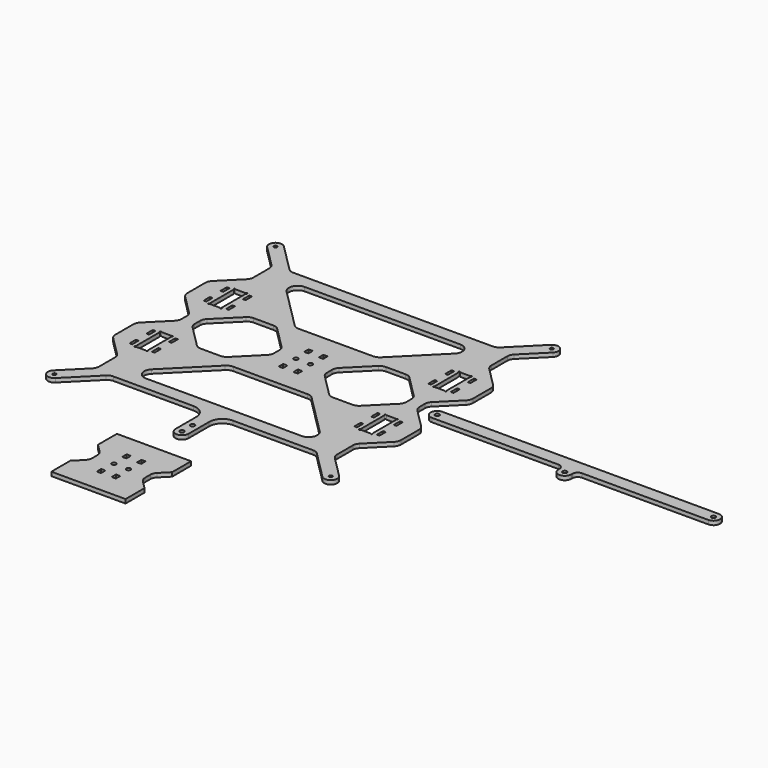
from build123d import *

# Parameters (mm, degrees)
F0_R     = 1.25
F0_W     = 2
F0_H     = 6
F0_R_2   = 1.6
F0_W_2   = 3.2
F0_H_2   = 4.2
F1_DEPTH = 3
F2_R     = 1.6
F3_DEPTH = 3
F6_R     = 1.25
F6_R_2   = 1.6
F6_W     = 2
F6_H     = 6
F7_DEPTH = 25


# Not quite as in the source:
# - ends of sketch curves that miss each other by under 0.0002 mm in the source are joined


with BuildPart() as f1:
    # F0 (on Top) → F1 (new body)
    with BuildSketch(Plane.XY):
        with BuildLine():
            ThreePointArc((-90.000032, 74.332551), (-90.4567550164, 72.0364496965), (-91.7573921058, 70.0899091058))
            Line((-91.7573921058, 70.0899091058), (-106.242677, 55.604628))
            ThreePointArc((-106.242677, 55.604628), (-107.5433139836, 53.6580873035), (-108.000037, 51.361986))
            Line((-108.000037, 51.361986), (-108.000037, 34.332561))
            ThreePointArc((-108.000037, 34.332561), (-107.5433139836, 32.0364596965), (-106.2426768942, 30.0899191058))
            Line((-106.2426768942, 30.0899191058), (-91.757392, 15.604638))
            ThreePointArc((-91.757392, 15.604638), (-90.4567550164, 13.6580973035), (-90.000032, 11.361996))
            Line((-90.000032, 11.361996), (-90.000032, 6.332547))
            ThreePointArc((-90.000032, 6.332547), (-90.4567550164, 4.0364456965), (-91.7573921058, 2.0899051058))
            Line((-91.7573921058, 2.0899051058), (-106.242677, -12.395376))
            ThreePointArc((-106.242677, -12.395376), (-107.5433139836, -14.3419166965), (-108.000037, -16.638018))
            Line((-108.000037, -16.638018), (-108.000037, -33.667443))
            ThreePointArc((-108.000037, -33.667443), (-107.5433139836, -35.9635443035), (-106.2426768942, -37.9100848942))
            Line((-106.2426768942, -37.9100848942), (-91.757392, -52.395366))
            ThreePointArc((-91.757392, -52.395366), (-90.4567550164, -54.3419066965), (-90.000032, -56.638008))
            Line((-90.000032, -56.638008), (-90.000032, -71.667432))
            ThreePointArc((-90.000032, -71.667432), (-90.4567550164, -73.9635333035), (-91.7573921058, -75.9100738942))
            Line((-91.7573921058, -75.9100738942), (-108.000037, -92.15271))
            ThreePointArc((-108.000037, -92.15271), (-108.0000399189, -99.1527094189), (-101.0000403311, -99.1527116689))
            Line((-101.0000403311, -99.1527116689), (-79.75736, -77.910043))
            ThreePointArc((-79.75736, -77.910043), (-77.8108196502, -76.6094067458), (-75.514719, -76.152684))
            Line((-75.514719, -76.152684), (-14.949747, -76.152684))
            ThreePointArc((-14.949747, -76.152684), (-7.8786791881, -79.0816161881), (-4.949747, -86.152684))
            Line((-4.949747, -86.152684), (-4.949747, -105.652688))
            ThreePointArc((-4.949747, -105.652688), (0, -110.602435), (4.949747, -105.652688))
            Line((4.949747, -105.652688), (4.949747, -86.152684))
            ThreePointArc((4.949747, -86.152684), (7.8786791881, -79.0816161881), (14.949747, -76.152684))
            Line((14.949747, -76.152684), (75.51472, -76.152684))
            ThreePointArc((75.51472, -76.152684), (77.8108203236, -76.6094066105), (79.7573603942, -77.9100426058))
            Line((79.7573603942, -77.9100426058), (101.00004, -99.152712))
            ThreePointArc((101.00004, -99.152712), (108.0000396689, -99.1527096689), (108.0000376689, -92.1527103311))
            Line((108.0000376689, -92.1527103311), (91.757322, -75.910003))
            ThreePointArc((91.757322, -75.910003), (90.4566842869, -73.9634619568), (89.999961, -71.66736))
            Line((89.999961, -71.66736), (89.999961, -56.638066))
            ThreePointArc((89.999961, -56.638066), (90.4566823928, -54.3419686162), (91.7573151058, -52.3954301058))
            Line((91.7573151058, -52.3954301058), (106.242579, -37.910128))
            ThreePointArc((106.242579, -37.910128), (107.5432106505, -35.9635916935), (107.999933, -33.667497))
            Line((107.999933, -33.667497), (107.999947, -16.638072))
            ThreePointArc((107.999947, -16.638072), (107.5432260227, -14.3419706193), (106.2425908942, -12.3954291058))
            Line((106.2425908942, -12.3954291058), (91.757319, 2.089867))
            ThreePointArc((91.757319, 2.089867), (90.4566842014, 4.036405465), (89.999962, 6.332504))
            Line((89.999962, 6.332504), (89.999961, 11.361951))
            ThreePointArc((89.999961, 11.361951), (90.4566847161, 13.6580559928), (91.7573251058, 15.6045988942))
            Line((91.7573251058, 15.6045988942), (106.242624, 30.089866))
            ThreePointArc((106.242624, 30.089866), (107.5432638092, 32.036405447), (107.999989, 34.332507))
            Line((107.999989, 34.332507), (108.000003, 51.361932))
            ThreePointArc((108.000003, 51.361932), (107.5432790462, 53.6580405668), (106.2426358942, 55.6045858942))
            Line((106.2426358942, 55.6045858942), (91.757328, 70.089844))
            ThreePointArc((91.757328, 70.089844), (90.4566857752, 72.0363864502), (89.999961, 74.332492))
            Line((89.999961, 74.332492), (89.999961, 89.361904))
            ThreePointArc((89.999961, 89.361904), (90.4566841517, 91.6580056302), (91.7573216058, 93.6045463942))
            Line((91.7573216058, 93.6045463942), (108.000038, 109.847254))
            ThreePointArc((108.000038, 109.847254), (108.0000394189, 116.8472529189), (101.0000403311, 116.8472546689))
            Line((101.0000403311, 116.8472546689), (79.757314, 95.60454))
            ThreePointArc((79.757314, 95.60454), (77.810773997, 94.3039044752), (75.514674, 93.847182))
            Line((75.514674, 93.847182), (-75.514673, 93.847182))
            ThreePointArc((-75.514673, 93.847182), (-77.8107733236, 94.3039046105), (-79.7573133942, 95.6045406058))
            Line((-79.7573133942, 95.6045406058), (-101.00004, 116.847255))
            ThreePointArc((-101.00004, 116.847255), (-108.0000396689, 116.8472526689), (-108.0000376689, 109.8472533311))
            Line((-108.0000376689, 109.8472533311), (-91.757392, 93.604617))
            ThreePointArc((-91.757392, 93.604617), (-90.4567550164, 91.6580763035), (-90.000032, 89.361975))
            Line((-90.000032, 89.361975), (-90.000032, 74.332551))
        make_face()
        with Locations((-104.500065, -95.652703)):
            Circle(F0_R, mode=Mode.SUBTRACT)
        with Locations((-93.500053, -34.152682)):
            Rectangle(F0_W, F0_H, mode=Mode.SUBTRACT)
        with BuildLine():
            Line((-81.366062, -38.202686), (-88.634023, -38.202686))
            ThreePointArc((-88.634023, -38.202686), (-88.8840230645, -38.2696733354), (-89.0670357764, -38.4526861291))
            ThreePointArc((-89.0670357764, -38.4526861291), (-89.8536023906, -38.5562393906), (-89.7500488709, -37.7696732236))
            ThreePointArc((-89.7500488709, -37.7696732236), (-89.5670362104, -37.586660848), (-89.500049, -37.336661))
            Line((-89.500049, -37.336661), (-89.500049, -14.96871))
            ThreePointArc((-89.500049, -14.96871), (-89.5670363354, -14.7187099355), (-89.7500491291, -14.5356972236))
            ThreePointArc((-89.7500491291, -14.5356972236), (-89.8536023906, -13.7491306094), (-89.0670362236, -13.8526841291))
            ThreePointArc((-89.0670362236, -13.8526841291), (-88.8840230645, -14.0356966646), (-88.634023, -14.102684))
            Line((-88.634023, -14.102684), (-81.366062, -14.102684))
            ThreePointArc((-81.366062, -14.102684), (-81.116062152, -14.0356967896), (-80.9330494736, -13.8526843039))
            ThreePointArc((-80.9330494736, -13.8526843039), (-80.1464836094, -13.7491306094), (-80.2500371291, -14.5356967764))
            ThreePointArc((-80.2500371291, -14.5356967764), (-80.4330496646, -14.7187099355), (-80.500037, -14.96871))
            Line((-80.500037, -14.96871), (-80.500037, -37.336661))
            ThreePointArc((-80.500037, -37.336661), (-80.4330497896, -37.586660848), (-80.2500373039, -37.7696735264))
            ThreePointArc((-80.2500373039, -37.7696735264), (-80.1464836094, -38.5562393906), (-80.9330497764, -38.4526858709))
            ThreePointArc((-80.9330497764, -38.4526858709), (-81.116062152, -38.2696732104), (-81.366062, -38.202686))
        make_face(mode=Mode.SUBTRACT)
        with Locations((-76.500053, -34.152682)):
            Rectangle(F0_W, F0_H, mode=Mode.SUBTRACT)
        with Locations((-93.500053, -18.152682)):
            Rectangle(F0_W, F0_H, mode=Mode.SUBTRACT)
        with Locations((-76.500053, -18.152682)):
            Rectangle(F0_W, F0_H, mode=Mode.SUBTRACT)
        Polygon((-4.000397, -5.25302), (-7.200397, -5.253021), (-7.200398, -1.053021), (-4.000398, -1.05302), align=None, mode=Mode.SUBTRACT)
        with Locations((0, -105.652688)):
            Circle(F0_R_2, mode=Mode.SUBTRACT)
        with Locations((0.000405, -95.653018)):
            Circle(F0_R_2, mode=Mode.SUBTRACT)
        with Locations((104.499935, -95.652703)):
            Circle(F0_R, mode=Mode.SUBTRACT)
        with BuildLine():
            Line((32.733092, -24.085784), (63.533098, -54.885791))
            ThreePointArc((63.533098, -54.885791), (64.9637982021, -62.0784045616), (58.866195, -66.152693))
            Line((58.866195, -66.152693), (-58.866183, -66.152693))
            ThreePointArc((-58.866183, -66.152693), (-64.9637860668, -62.0784048882), (-63.5330863416, -54.8857916584))
            Line((-63.5330863416, -54.8857916584), (-32.733081, -24.085784))
            ThreePointArc((-32.733081, -24.085784), (-30.5918868882, -22.6550849332), (-28.066177, -22.15269))
            Line((-28.066177, -22.15269), (28.066188, -22.15269))
            ThreePointArc((28.066188, -22.15269), (30.5918978882, -22.6550849332), (32.733092, -24.085784))
        make_face(mode=Mode.SUBTRACT)
        with Locations((5.600405, -3.153018)):
            Rectangle(F0_W_2, F0_H_2, mode=Mode.SUBTRACT)
        with Locations((76.499864, -34.152719)):
            Rectangle(F0_W, F0_H, mode=Mode.SUBTRACT)
        with Locations((93.499864, -34.152719)):
            Rectangle(F0_W, F0_H, mode=Mode.SUBTRACT)
        with BuildLine():
            Line((89.499899, -14.968747), (89.499881, -37.336698))
            ThreePointArc((89.499881, -37.336698), (89.5668683354, -37.5866980645), (89.7498811291, -37.7697107764))
            ThreePointArc((89.7498811291, -37.7697107764), (89.8534330844, -38.5562766968), (89.0668674736, -38.4527233039))
            ThreePointArc((89.0668674736, -38.4527233039), (88.8838550645, -38.2697103354), (88.633855, -38.202723))
            Line((88.633855, -38.202723), (81.365894, -38.202723))
            ThreePointArc((81.365894, -38.202723), (81.1158939355, -38.2697103354), (80.9328812236, -38.4527231291))
            ThreePointArc((80.9328812236, -38.4527231291), (80.1463143032, -38.5562760844), (80.2498688791, -37.7697097906))
            ThreePointArc((80.2498688791, -37.7697097906), (80.4328817896, -37.586697848), (80.499869, -37.336698))
            Line((80.499869, -37.336698), (80.499887, -14.968747))
            ThreePointArc((80.499887, -14.968747), (80.4328996646, -14.7187469355), (80.2498868709, -14.5357342236))
            ThreePointArc((80.2498868709, -14.5357342236), (80.1463349156, -13.7491683032), (80.9329005264, -13.8527216961))
            ThreePointArc((80.9329005264, -13.8527216961), (81.1159129355, -14.0357346646), (81.365913, -14.102722))
            Line((81.365913, -14.102722), (88.633874, -14.102722))
            ThreePointArc((88.633874, -14.102722), (88.8838740645, -14.0357346646), (89.0668867764, -13.8527218709))
            ThreePointArc((89.0668867764, -13.8527218709), (89.8534523906, -13.7491686094), (89.7498993039, -14.5357345264))
            ThreePointArc((89.7498993039, -14.5357345264), (89.5668863354, -14.7187469355), (89.499899, -14.968747))
        make_face(mode=Mode.SUBTRACT)
        with Locations((76.499864, -18.152719)):
            Rectangle(F0_W, F0_H, mode=Mode.SUBTRACT)
        with Locations((93.499864, -18.152719)):
            Rectangle(F0_W, F0_H, mode=Mode.SUBTRACT)
        with Locations((-93.500075, 35.847342)):
            Rectangle(F0_W, F0_H, mode=Mode.SUBTRACT)
        with BuildLine():
            Line((-81.366085, 31.797338), (-88.634046, 31.797338))
            ThreePointArc((-88.634046, 31.797338), (-88.8840460645, 31.7303506646), (-89.0670587764, 31.5473378709))
            ThreePointArc((-89.0670587764, 31.5473378709), (-89.8536245674, 31.4437847862), (-89.7500708709, 32.2303507764))
            ThreePointArc((-89.7500708709, 32.2303507764), (-89.5670582104, 32.413363152), (-89.500071, 32.663363))
            Line((-89.500071, 32.663363), (-89.500071, 55.031314))
            ThreePointArc((-89.500071, 55.031314), (-89.5670583354, 55.2813140645), (-89.7500711291, 55.4643267764))
            ThreePointArc((-89.7500711291, 55.4643267764), (-89.8536245674, 56.2508932138), (-89.0670584736, 56.1473403039))
            ThreePointArc((-89.0670584736, 56.1473403039), (-88.8840460645, 55.9643273354), (-88.634046, 55.89734))
            Line((-88.634046, 55.89734), (-81.366085, 55.89734))
            ThreePointArc((-81.366085, 55.89734), (-81.1160849355, 55.9643273354), (-80.9330722236, 56.1473401291))
            ThreePointArc((-80.9330722236, 56.1473401291), (-80.1465064326, 56.2508932138), (-80.2500601291, 55.4643272236))
            ThreePointArc((-80.2500601291, 55.4643272236), (-80.4330726646, 55.2813140645), (-80.50006, 55.031314))
            Line((-80.50006, 55.031314), (-80.50006, 32.663363))
            ThreePointArc((-80.50006, 32.663363), (-80.4330727896, 32.413363152), (-80.2500603039, 32.2303504736))
            ThreePointArc((-80.2500603039, 32.2303504736), (-80.1465064326, 31.4437847862), (-80.9330725264, 31.5473376961))
            ThreePointArc((-80.9330725264, 31.5473376961), (-81.1160849355, 31.7303506646), (-81.366085, 31.797338))
        make_face(mode=Mode.SUBTRACT)
        with Locations((-93.500075, 51.847342)):
            Rectangle(F0_W, F0_H, mode=Mode.SUBTRACT)
        with Locations((-76.500075, 35.847342)):
            Rectangle(F0_W, F0_H, mode=Mode.SUBTRACT)
        with Locations((-76.500075, 51.847342)):
            Rectangle(F0_W, F0_H, mode=Mode.SUBTRACT)
        with BuildLine():
            Line((-78.242655, 15.604638), (-61.757389, 32.089899))
            ThreePointArc((-61.757389, 32.089899), (-59.8108486502, 33.3905352542), (-57.514748, 33.847258))
            Line((-57.514748, 33.847258), (-42.485324, 33.847258))
            ThreePointArc((-42.485324, 33.847258), (-40.1892236764, 33.3905353895), (-38.2426836058, 32.0898993942))
            Line((-38.2426836058, 32.0898993942), (-21.757418, 15.604638))
            ThreePointArc((-21.757418, 15.604638), (-20.4567810164, 13.6580973035), (-20.000058, 11.361996))
            Line((-20.000058, 11.361996), (-20.000058, 6.332547))
            ThreePointArc((-20.000058, 6.332547), (-20.4567810164, 4.0364456965), (-21.7574181058, 2.0899051058))
            Line((-21.7574181058, 2.0899051058), (-38.242684, -14.395356))
            ThreePointArc((-38.242684, -14.395356), (-40.1892236764, -15.6959923895), (-42.485324, -16.152715))
            Line((-42.485324, -16.152715), (-57.514748, -16.152715))
            ThreePointArc((-57.514748, -16.152715), (-59.8108486502, -15.6959922542), (-61.7573888942, -14.3953558942))
            Line((-61.7573888942, -14.3953558942), (-78.242655, 2.089905))
            ThreePointArc((-78.242655, 2.089905), (-79.5432919836, 4.0364456965), (-80.000015, 6.332547))
            Line((-80.000015, 6.332547), (-80.000015, 11.361996))
            ThreePointArc((-80.000015, 11.361996), (-79.5432919836, 13.6580973035), (-78.242655, 15.604638))
        make_face(mode=Mode.SUBTRACT)
        with Locations((-5.499595, 8.846982)):
            Circle(F0_R_2, mode=Mode.SUBTRACT)
        Polygon((-4.000398, 18.747655), (-7.200398, 18.747656), (-7.200397, 22.947656), (-4.000397, 22.947655), align=None, mode=Mode.SUBTRACT)
        with Locations((-104.500065, 113.347297)):
            Circle(F0_R, mode=Mode.SUBTRACT)
        with BuildLine():
            Line((63.533091, 72.580426), (32.733084, 41.780419))
            ThreePointArc((32.733084, 41.780419), (30.5918905616, 40.3497197979), (28.066181, 39.847325))
            Line((28.066181, 39.847325), (-28.066184, 39.847325))
            ThreePointArc((-28.066184, 39.847325), (-30.5918938882, 40.3497199332), (-32.7330873416, 41.7804196584))
            Line((-32.7330873416, 41.7804196584), (-63.533095, 72.580426))
            ThreePointArc((-63.533095, 72.580426), (-64.9637940668, 79.7730398882), (-58.866191, 83.847328))
            Line((-58.866191, 83.847328), (58.866187, 83.847328))
            ThreePointArc((58.866187, 83.847328), (64.9637900668, 79.7730398882), (63.533091, 72.580426))
        make_face(mode=Mode.SUBTRACT)
        with Locations((5.500405, 8.846982)):
            Circle(F0_R_2, mode=Mode.SUBTRACT)
        with Locations((5.600405, 20.847653)):
            Rectangle(F0_W_2, F0_H_2, mode=Mode.SUBTRACT)
        with BuildLine():
            Line((38.242594, -14.395352), (21.757344, 2.089925))
            ThreePointArc((21.757344, 2.089925), (20.456709934, 4.0364643096), (19.999988, 6.332563))
            Line((19.999988, 6.332563), (19.999988, 11.362012))
            ThreePointArc((19.999988, 11.362012), (20.456712234, 13.6581162433), (21.7573526058, 15.6046583942))
            Line((21.7573526058, 15.6046583942), (38.242634, 32.089903))
            ThreePointArc((38.242634, 32.089903), (40.1891729629, 33.3905363366), (42.485271, 33.847258))
            Line((42.485271, 33.847258), (57.514695, 33.847258))
            ThreePointArc((57.514695, 33.847258), (59.8107979367, 33.3905343072), (61.7573393942, 32.0898953942))
            Line((61.7573393942, 32.0898953942), (78.242589, 15.604618))
            ThreePointArc((78.242589, 15.604618), (79.543223066, 13.6580786904), (79.999945, 11.36198))
            Line((79.999945, 11.36198), (79.999945, 6.332531))
            ThreePointArc((79.999945, 6.332531), (79.5432209013, 4.0364270834), (78.2425808942, 2.0898851058))
            Line((78.2425808942, 2.0898851058), (61.757299, -14.39536))
            ThreePointArc((61.757299, -14.39536), (59.8107607105, -15.6959934719), (57.514663, -16.152715))
            Line((57.514663, -16.152715), (42.485239, -16.152715))
            ThreePointArc((42.485239, -16.152715), (40.1891357366, -15.6959911719), (38.242594, -14.395352))
        make_face(mode=Mode.SUBTRACT)
        with Locations((76.499945, 35.847305)):
            Rectangle(F0_W, F0_H, mode=Mode.SUBTRACT)
        with Locations((76.499945, 51.847305)):
            Rectangle(F0_W, F0_H, mode=Mode.SUBTRACT)
        with Locations((93.499945, 35.847305)):
            Rectangle(F0_W, F0_H, mode=Mode.SUBTRACT)
        with BuildLine():
            Line((89.499979, 55.031277), (89.499961, 32.663326))
            ThreePointArc((89.499961, 32.663326), (89.5669483354, 32.4133259355), (89.7499611291, 32.2303132236))
            ThreePointArc((89.7499611291, 32.2303132236), (89.8535142138, 31.4437474326), (89.0669482236, 31.5473011291))
            ThreePointArc((89.0669482236, 31.5473011291), (88.8839350645, 31.7303136646), (88.633935, 31.797301))
            Line((88.633935, 31.797301), (81.365974, 31.797301))
            ThreePointArc((81.365974, 31.797301), (81.115974152, 31.7303137896), (80.9329614736, 31.5473013039))
            ThreePointArc((80.9329614736, 31.5473013039), (80.1463956094, 31.4437476094), (80.2499491291, 32.2303137764))
            ThreePointArc((80.2499491291, 32.2303137764), (80.4329625731, 32.413325777), (80.49995, 32.663326))
            Line((80.49995, 32.663326), (80.499967, 55.031277))
            ThreePointArc((80.499967, 55.031277), (80.4329798811, 55.2812766895), (80.2499676209, 55.4642893434))
            ThreePointArc((80.2499676209, 55.4642893434), (80.1464147862, 56.2508555674), (80.9329807764, 56.1473018709))
            ThreePointArc((80.9329807764, 56.1473018709), (81.1159939355, 55.9642893354), (81.365994, 55.897302))
            Line((81.365994, 55.897302), (88.633955, 55.897302))
            ThreePointArc((88.633955, 55.897302), (88.883954848, 55.9642892104), (89.0669675264, 56.1473016961))
            ThreePointArc((89.0669675264, 56.1473016961), (89.8535332138, 56.2508555674), (89.7499803039, 55.4642894736))
            ThreePointArc((89.7499803039, 55.4642894736), (89.5669665519, 55.2812774395), (89.499979, 55.031277))
        make_face(mode=Mode.SUBTRACT)
        with Locations((93.499945, 51.847305)):
            Rectangle(F0_W, F0_H, mode=Mode.SUBTRACT)
        with Locations((104.499935, 113.347297)):
            Circle(F0_R, mode=Mode.SUBTRACT)
    extrude(amount=F1_DEPTH)


with BuildPart() as f3:
    # F2 (on Top) → F3 (new body)
    with BuildSketch(Plane.XY):
        with BuildLine():
            Line((8.949747, 0.05025), (104.500004, 0.050253))
            ThreePointArc((104.500004, 0.050253), (109.449747, 5), (104.500004, 9.949747))
            Line((104.500004, 9.949747), (-104.500004, 9.949747))
            ThreePointArc((-104.500004, 9.949747), (-109.449747, 5), (-104.500004, 0.050253))
            Line((-104.500004, 0.050253), (-8.949747, 0.050255))
            ThreePointArc((-8.949747, 0.050255), (-6.1213198753, -1.1213178753), (-4.949747, -3.949745))
            Line((-4.949747, -3.949745), (-4.949747, -5.000004))
            ThreePointArc((-4.949747, -5.000004), (0, -9.949747), (4.949747, -5.000004))
            Line((4.949747, -5.000004), (4.949747, -3.949751))
            ThreePointArc((4.949747, -3.949751), (6.1213195217, -1.1213232288), (8.949747, 0.05025))
        make_face()
        with Locations((0, -5)):
            Circle(F2_R, mode=Mode.SUBTRACT)
        with Locations((-104.5, 5)):
            Circle(F2_R, mode=Mode.SUBTRACT)
        with Locations((104.5, 5)):
            Circle(F2_R, mode=Mode.SUBTRACT)
    extrude(amount=F3_DEPTH)


with BuildPart() as f3_1:
    # F4: moved
    add(f3.part.moved(Location((209.000008, 0, 0))))


with BuildPart() as f5_1:
    # F5: copy of F1
    add(f1.part.moved(Location((0, -172, 0))))

    # F6 (on face) → F7 (cut)
    with BuildSketch(Plane.XY.offset(3)):
        with BuildLine():
            Line((-90.000032, -82.638025), (-90.000032, -97.667449))
            ThreePointArc((-90.000032, -97.667449), (-90.4567550164, -99.9635503035), (-91.7573921058, -101.9100908942))
            Line((-91.7573921058, -101.9100908942), (-106.242677, -116.395372))
            ThreePointArc((-106.242677, -116.395372), (-107.543313978, -118.3419126827), (-108.000037, -120.638014))
            Line((-108.000037, -120.638014), (-108.000037, -137.667439))
            ThreePointArc((-108.000037, -137.667439), (-107.5433139836, -139.9635403035), (-106.2426768942, -141.9100808942))
            Line((-106.2426768942, -141.9100808942), (-91.757392, -156.395362))
            ThreePointArc((-91.757392, -156.395362), (-90.456755022, -158.3419026827), (-90.000032, -160.638004))
            Line((-90.000032, -160.638004), (-90.000032, -165.667453))
            ThreePointArc((-90.000032, -165.667453), (-90.4567550164, -167.9635543035), (-91.7573921058, -169.9100948942))
            Line((-91.7573921058, -169.9100948942), (-106.242677, -184.395376))
            ThreePointArc((-106.242677, -184.395376), (-107.543313978, -186.3419166827), (-108.000037, -188.638018))
            Line((-108.000037, -188.638018), (-108.000037, -205.667443))
            ThreePointArc((-108.000037, -205.667443), (-107.5433139836, -207.9635443035), (-106.2426768942, -209.9100848942))
            Line((-106.2426768942, -209.9100848942), (-91.757392, -224.395366))
            ThreePointArc((-91.757392, -224.395366), (-90.456755022, -226.3419066827), (-90.000032, -228.638008))
            Line((-90.000032, -228.638008), (-90.000032, -243.667432))
            ThreePointArc((-90.000032, -243.667432), (-90.4567550164, -245.9635333035), (-91.7573921058, -247.9100738942))
            Line((-91.7573921058, -247.9100738942), (-108.000037, -264.15271))
            ThreePointArc((-108.000037, -264.15271), (-108.0000398344, -271.1527095033), (-101.0000403311, -271.1527116689))
            Line((-101.0000403311, -271.1527116689), (-79.75736, -249.910043))
            ThreePointArc((-79.75736, -249.910043), (-77.810819664, -248.6094067514), (-75.514719, -248.152684))
            Line((-75.514719, -248.152684), (-14.949747, -248.152684))
            ThreePointArc((-14.949747, -248.152684), (-7.8786791881, -251.0816161881), (-4.949747, -258.152684))
            Line((-4.949747, -258.152684), (-4.949747, -277.652688))
            ThreePointArc((-4.949747, -277.652688), (0, -282.602435), (4.949747, -277.652688))
            Line((4.949747, -277.652688), (4.949747, -258.152684))
            ThreePointArc((4.949747, -258.152684), (7.8786791881, -251.0816161881), (14.949747, -248.152684))
            Line((14.949747, -248.152684), (75.51472, -248.152684))
            ThreePointArc((75.51472, -248.152684), (77.8108203236, -248.6094066105), (79.7573603942, -249.9100426058))
            Line((79.7573603942, -249.9100426058), (101.00004, -271.152712))
            ThreePointArc((101.00004, -271.152712), (108.0000395033, -271.1527098344), (108.0000376689, -264.1527103311))
            Line((108.0000376689, -264.1527103311), (91.757322, -247.910003))
            ThreePointArc((91.757322, -247.910003), (90.4566842926, -245.9634619705), (89.999961, -243.66736))
            Line((89.999961, -243.66736), (89.999961, -228.638066))
            ThreePointArc((89.999961, -228.638066), (90.4566823928, -226.3419686162), (91.7573151058, -224.3954301058))
            Line((91.7573151058, -224.3954301058), (106.242579, -209.910128))
            ThreePointArc((106.242579, -209.910128), (107.5432106448, -207.9635917073), (107.999933, -205.667497))
            Line((107.999933, -205.667497), (107.999947, -188.638072))
            ThreePointArc((107.999947, -188.638072), (107.5432260227, -186.3419706193), (106.2425908942, -184.3954291058))
            Line((106.2425908942, -184.3954291058), (91.757319, -169.910133))
            ThreePointArc((91.757319, -169.910133), (90.4566841691, -167.9635944569), (89.999962, -165.667496))
            Line((89.999962, -165.667496), (89.999961, -160.638049))
            ThreePointArc((89.999961, -160.638049), (90.4566847161, -158.3419440072), (91.7573251058, -156.3954011058))
            Line((91.7573251058, -156.3954011058), (106.242624, -141.910134))
            ThreePointArc((106.242624, -141.910134), (107.5432638305, -139.9635945018), (107.999989, -137.667493))
            Line((107.999989, -137.667493), (108.000003, -120.638068))
            ThreePointArc((108.000003, -120.638068), (107.5432790462, -118.3419594332), (106.2426358942, -116.3954141058))
            Line((106.2426358942, -116.3954141058), (91.757328, -101.910156))
            ThreePointArc((91.757328, -101.910156), (90.456685754, -99.9636134986), (89.999961, -97.667508))
            Line((89.999961, -97.667508), (89.999961, -82.638096))
            ThreePointArc((89.999961, -82.638096), (90.4566841517, -80.3419943698), (91.7573216058, -78.3954536058))
            Line((91.7573216058, -78.3954536058), (108.000038, -62.152746))
            ThreePointArc((108.000038, -62.152746), (108.0000393344, -55.1527469967), (101.0000403311, -55.1527453311))
            Line((101.0000403311, -55.1527453311), (79.757314, -76.39546))
            ThreePointArc((79.757314, -76.39546), (77.8107740107, -77.6960955192), (75.514674, -78.152818))
            Line((75.514674, -78.152818), (-75.514673, -78.152818))
            ThreePointArc((-75.514673, -78.152818), (-77.8107733236, -77.6960953895), (-79.7573133942, -76.3954593942))
            Line((-79.7573133942, -76.3954593942), (-101.00004, -55.152745))
            ThreePointArc((-101.00004, -55.152745), (-108.0000395033, -55.1527471656), (-108.0000376689, -62.1527466689))
            Line((-108.0000376689, -62.1527466689), (-91.757392, -78.395383))
            ThreePointArc((-91.757392, -78.395383), (-90.456755022, -80.3419236827), (-90.000032, -82.638025))
        make_face()
        with Locations((-104.500065, -267.652703)):
            Circle(F6_R, mode=Mode.SUBTRACT)
        with Locations((0, -277.652688)):
            Circle(F6_R_2, mode=Mode.SUBTRACT)
        with Locations((-93.500053, -206.152682)):
            Rectangle(F6_W, F6_H, mode=Mode.SUBTRACT)
        with BuildLine():
            ThreePointArc((-80.2500373039, -209.7696735264), (-80.1464837705, -210.5562395517), (-80.9330497764, -210.4526858709))
            ThreePointArc((-80.9330497764, -210.4526858709), (-81.1160621925, -210.2696731869), (-81.366062, -210.202686))
            Line((-81.366062, -210.202686), (-88.634023, -210.202686))
            ThreePointArc((-88.634023, -210.202686), (-88.8840230645, -210.2696733354), (-89.0670357764, -210.4526861291))
            ThreePointArc((-89.0670357764, -210.4526861291), (-89.8536021527, -210.5562396285), (-89.7500488709, -209.7696732236))
            ThreePointArc((-89.7500488709, -209.7696732236), (-89.5670361869, -209.5866608075), (-89.500049, -209.336661))
            Line((-89.500049, -209.336661), (-89.500049, -186.96871))
            ThreePointArc((-89.500049, -186.96871), (-89.5670363354, -186.7187099355), (-89.7500491291, -186.5356972236))
            ThreePointArc((-89.7500491291, -186.5356972236), (-89.8536026285, -185.7491308473), (-89.0670362236, -185.8526841291))
            ThreePointArc((-89.0670362236, -185.8526841291), (-88.8840231245, -186.03569663), (-88.634023, -186.102684))
            Line((-88.634023, -186.102684), (-81.366062, -186.102684))
            ThreePointArc((-81.366062, -186.102684), (-81.116062152, -186.0356967896), (-80.9330494736, -185.8526843039))
            ThreePointArc((-80.9330494736, -185.8526843039), (-80.1464834483, -185.7491307705), (-80.2500371291, -186.5356967764))
            ThreePointArc((-80.2500371291, -186.5356967764), (-80.43304963, -186.7187098755), (-80.500037, -186.96871))
            Line((-80.500037, -186.96871), (-80.500037, -209.336661))
            ThreePointArc((-80.500037, -209.336661), (-80.4330497896, -209.586660848), (-80.2500373039, -209.7696735264))
        make_face(mode=Mode.SUBTRACT)
        with Locations((-76.500053, -206.152682)):
            Rectangle(F6_W, F6_H, mode=Mode.SUBTRACT)
        with Locations((-93.500053, -190.152682)):
            Rectangle(F6_W, F6_H, mode=Mode.SUBTRACT)
        with Locations((-76.500053, -190.152682)):
            Rectangle(F6_W, F6_H, mode=Mode.SUBTRACT)
        with Locations((0.000405, -267.653018)):
            Circle(F6_R_2, mode=Mode.SUBTRACT)
        with Locations((104.499935, -267.652703)):
            Circle(F6_R, mode=Mode.SUBTRACT)
        with Locations((76.499864, -206.152719)):
            Rectangle(F6_W, F6_H, mode=Mode.SUBTRACT)
        with Locations((93.499864, -206.152719)):
            Rectangle(F6_W, F6_H, mode=Mode.SUBTRACT)
        with BuildLine():
            ThreePointArc((80.9329005264, -185.8527216961), (81.115912976, -186.0357346881), (81.365913, -186.102722))
            Line((81.365913, -186.102722), (88.633874, -186.102722))
            ThreePointArc((88.633874, -186.102722), (88.8838740645, -186.0357346646), (89.0668867764, -185.8527218709))
            ThreePointArc((89.0668867764, -185.8527218709), (89.8534525517, -185.7491687705), (89.7498993039, -186.5357345264))
            ThreePointArc((89.7498993039, -186.5357345264), (89.5668863119, -186.718746976), (89.499899, -186.968747))
            Line((89.499899, -186.968747), (89.499881, -209.336698))
            ThreePointArc((89.499881, -209.336698), (89.5668683354, -209.5866980645), (89.7498811291, -209.7697107764))
            ThreePointArc((89.7498811291, -209.7697107764), (89.8534331537, -210.5562766275), (89.0668674736, -210.4527233039))
            ThreePointArc((89.0668674736, -210.4527233039), (88.883855024, -210.2697103119), (88.633855, -210.202723))
            Line((88.633855, -210.202723), (81.365894, -210.202723))
            ThreePointArc((81.365894, -210.202723), (81.1158939355, -210.2697103354), (80.9328812236, -210.4527231291))
            ThreePointArc((80.9328812236, -210.4527231291), (80.1463145411, -210.5562763223), (80.2498688791, -209.7697097906))
            ThreePointArc((80.2498688791, -209.7697097906), (80.4328818465, -209.5866977495), (80.499869, -209.336698))
            Line((80.499869, -209.336698), (80.499887, -186.968747))
            ThreePointArc((80.499887, -186.968747), (80.4328996646, -186.7187469355), (80.2498868709, -186.5357342236))
            ThreePointArc((80.2498868709, -186.5357342236), (80.1463348463, -185.7491683725), (80.9329005264, -185.8527216961))
        make_face(mode=Mode.SUBTRACT)
        with Locations((76.499864, -190.152719)):
            Rectangle(F6_W, F6_H, mode=Mode.SUBTRACT)
        with Locations((93.499864, -190.152719)):
            Rectangle(F6_W, F6_H, mode=Mode.SUBTRACT)
        with Locations((-93.500075, -136.152658)):
            Rectangle(F6_W, F6_H, mode=Mode.SUBTRACT)
        with BuildLine():
            ThreePointArc((-80.9330725264, -140.4526623039), (-81.116084976, -140.2696493119), (-81.366085, -140.202662))
            Line((-81.366085, -140.202662), (-88.634046, -140.202662))
            ThreePointArc((-88.634046, -140.202662), (-88.8840460645, -140.2696493354), (-89.0670587764, -140.4526621291))
            ThreePointArc((-89.0670587764, -140.4526621291), (-89.8536247285, -140.5562150527), (-89.7500708709, -139.7696492236))
            ThreePointArc((-89.7500708709, -139.7696492236), (-89.5670581869, -139.5866368075), (-89.500071, -139.336637))
            Line((-89.500071, -139.336637), (-89.500071, -116.968686))
            ThreePointArc((-89.500071, -116.968686), (-89.5670583354, -116.7186859355), (-89.7500711291, -116.5356732236))
            ThreePointArc((-89.7500711291, -116.5356732236), (-89.8536248053, -115.7491070241), (-89.0670584736, -115.8526596961))
            ThreePointArc((-89.0670584736, -115.8526596961), (-88.884046024, -116.0356726881), (-88.634046, -116.10266))
            Line((-88.634046, -116.10266), (-81.366085, -116.10266))
            ThreePointArc((-81.366085, -116.10266), (-81.1160849355, -116.0356726646), (-80.9330722236, -115.8526598709))
            ThreePointArc((-80.9330722236, -115.8526598709), (-80.1465062715, -115.7491069473), (-80.2500601291, -116.5356727764))
            ThreePointArc((-80.2500601291, -116.5356727764), (-80.43307263, -116.7186858755), (-80.50006, -116.968686))
            Line((-80.50006, -116.968686), (-80.50006, -139.336637))
            ThreePointArc((-80.50006, -139.336637), (-80.4330727896, -139.586636848), (-80.2500603039, -139.7696495264))
            ThreePointArc((-80.2500603039, -139.7696495264), (-80.1465065938, -140.5562153749), (-80.9330725264, -140.4526623039))
        make_face(mode=Mode.SUBTRACT)
        with Locations((-93.500075, -120.152658)):
            Rectangle(F6_W, F6_H, mode=Mode.SUBTRACT)
        with Locations((-76.500075, -136.152658)):
            Rectangle(F6_W, F6_H, mode=Mode.SUBTRACT)
        with Locations((-76.500075, -120.152658)):
            Rectangle(F6_W, F6_H, mode=Mode.SUBTRACT)
        with BuildLine():
            Line((-28.066184, -150.0865976117), (-28.066184, -132.152675))
            ThreePointArc((-28.066184, -132.152675), (-30.5918938882, -131.6502800668), (-32.7330873416, -130.2195803416))
            Line((-32.7330873416, -130.2195803416), (-63.533095, -99.419574))
            ThreePointArc((-63.533095, -99.419574), (-64.9637941859, -92.2269603991), (-58.866191, -88.152672))
            Line((-58.866191, -88.152672), (58.866187, -88.152672))
            ThreePointArc((58.866187, -88.152672), (64.9637901859, -92.2269603991), (63.533091, -99.419574))
            Line((63.533091, -99.419574), (32.733084, -130.219581))
            ThreePointArc((32.733084, -130.219581), (30.5918905822, -131.6502801936), (28.066181, -132.152675))
            Line((28.066181, -132.152675), (28.066188, -150.0865202903))
            Line((28.066188, -150.0865202903), (38.242634, -139.910097))
            ThreePointArc((38.242634, -139.910097), (40.1891729491, -138.6094636691), (42.485271, -138.152742))
            Line((42.485271, -138.152742), (57.514695, -138.152742))
            ThreePointArc((57.514695, -138.152742), (59.8107979367, -138.6094656928), (61.7573393942, -139.9101046058))
            Line((61.7573393942, -139.9101046058), (78.242589, -156.395382))
            ThreePointArc((78.242589, -156.395382), (79.5432230603, -158.3419212959), (79.999945, -160.63802))
            Line((79.999945, -160.63802), (79.999945, -165.667469))
            ThreePointArc((79.999945, -165.667469), (79.5432209013, -167.9635729166), (78.2425808942, -169.9101148942))
            Line((78.2425808942, -169.9101148942), (61.757299, -186.39536))
            ThreePointArc((61.757299, -186.39536), (59.8107606592, -187.6959934932), (57.514663, -188.152715))
            Line((57.514663, -188.152715), (42.485239, -188.152715))
            ThreePointArc((42.485239, -188.152715), (40.1891357229, -187.6959911662), (38.242594, -186.395352))
            Line((38.242594, -186.395352), (28.066188, -176.2189293328))
            Line((28.066188, -176.2189293328), (28.066188, -194.15269))
            ThreePointArc((28.066188, -194.15269), (30.5918979738, -194.6550849686), (32.733092, -196.085784))
            Line((32.733092, -196.085784), (63.533098, -226.885791))
            ThreePointArc((63.533098, -226.885791), (64.9637982308, -234.0784044925), (58.866195, -238.152693))
            Line((58.866195, -238.152693), (-58.866183, -238.152693))
            ThreePointArc((-58.866183, -238.152693), (-64.9637860668, -234.0784048882), (-63.5330863416, -226.8857916584))
            Line((-63.5330863416, -226.8857916584), (-32.733081, -196.085784))
            ThreePointArc((-32.733081, -196.085784), (-30.5918869738, -194.6550849686), (-28.066177, -194.15269))
            Line((-28.066177, -194.15269), (-28.066184, -176.218858956))
            Line((-28.066184, -176.218858956), (-38.242684, -186.395356))
            ThreePointArc((-38.242684, -186.395356), (-40.1892237276, -187.6959924108), (-42.485324, -188.152715))
            Line((-42.485324, -188.152715), (-57.514748, -188.152715))
            ThreePointArc((-57.514748, -188.152715), (-59.8108486502, -187.6959922542), (-61.7573888942, -186.3953558942))
            Line((-61.7573888942, -186.3953558942), (-78.242655, -169.910095))
            ThreePointArc((-78.242655, -169.910095), (-79.543291978, -167.9635543173), (-80.000015, -165.667453))
            Line((-80.000015, -165.667453), (-80.000015, -160.638004))
            ThreePointArc((-80.000015, -160.638004), (-79.543291978, -158.3419026827), (-78.242655, -156.395362))
            Line((-78.242655, -156.395362), (-61.757389, -139.910101))
            ThreePointArc((-61.757389, -139.910101), (-59.810848664, -138.6094647514), (-57.514748, -138.152742))
            Line((-57.514748, -138.152742), (-42.485324, -138.152742))
            ThreePointArc((-42.485324, -138.152742), (-40.1892236764, -138.6094646105), (-38.2426836058, -139.9101006058))
            Line((-38.2426836058, -139.9101006058), (-28.066184, -150.0865976117))
        make_face(mode=Mode.SUBTRACT)
        with Locations((-104.500065, -58.652703)):
            Circle(F6_R, mode=Mode.SUBTRACT)
        with Locations((76.499945, -136.152695)):
            Rectangle(F6_W, F6_H, mode=Mode.SUBTRACT)
        with Locations((76.499945, -120.152695)):
            Rectangle(F6_W, F6_H, mode=Mode.SUBTRACT)
        with Locations((93.499945, -136.152695)):
            Rectangle(F6_W, F6_H, mode=Mode.SUBTRACT)
        with BuildLine():
            ThreePointArc((80.9329807764, -115.8526981291), (81.1159938755, -116.03571063), (81.365994, -116.102698))
            Line((81.365994, -116.102698), (88.633955, -116.102698))
            ThreePointArc((88.633955, -116.102698), (88.883954848, -116.0357107896), (89.0669675264, -115.8526983039))
            ThreePointArc((89.0669675264, -115.8526983039), (89.8535333749, -115.7491445938), (89.7499803039, -116.5357105264))
            ThreePointArc((89.7499803039, -116.5357105264), (89.566966495, -116.718722659), (89.499979, -116.968723))
            Line((89.499979, -116.968723), (89.499961, -139.336674))
            ThreePointArc((89.499961, -139.336674), (89.5669483354, -139.5866740645), (89.7499611291, -139.7696867764))
            ThreePointArc((89.7499611291, -139.7696867764), (89.8535140527, -140.5562527285), (89.0669482236, -140.4526988709))
            ThreePointArc((89.0669482236, -140.4526988709), (88.8839351245, -140.26968637), (88.633935, -140.202699))
            Line((88.633935, -140.202699), (81.365974, -140.202699))
            ThreePointArc((81.365974, -140.202699), (81.115974152, -140.2696862104), (80.9329614736, -140.4526986961))
            ThreePointArc((80.9329614736, -140.4526986961), (80.1463954483, -140.5562522295), (80.2499491291, -139.7696862236))
            ThreePointArc((80.2499491291, -139.7696862236), (80.43296263, -139.5866741245), (80.49995, -139.336674))
            Line((80.49995, -139.336674), (80.499967, -116.968723))
            ThreePointArc((80.499967, -116.968723), (80.4329798811, -116.7187233105), (80.2499676209, -116.5357106566))
            ThreePointArc((80.2499676209, -116.5357106566), (80.1464147169, -115.7491445019), (80.9329807764, -115.8526981291))
        make_face(mode=Mode.SUBTRACT)
        with Locations((93.499945, -120.152695)):
            Rectangle(F6_W, F6_H, mode=Mode.SUBTRACT)
        with Locations((104.499935, -58.652703)):
            Circle(F6_R, mode=Mode.SUBTRACT)
        with Locations((-104.500065, -95.652703)):
            Circle(F6_R)
    extrude(amount=-F7_DEPTH, mode=Mode.SUBTRACT)


solid = Compound([f1.part, f3_1.part, f5_1.part])
